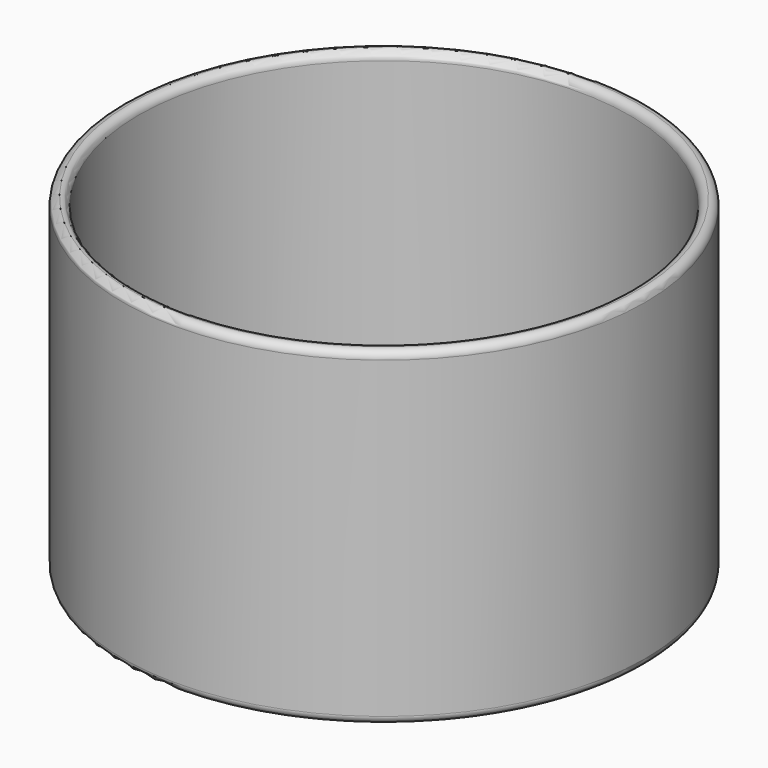
from build123d import *

# Parameters (mm, degrees)
F0_W = 42.2452799976
F0_H = 53.2546564937
F2_T = -2.54
F3_R = 1.26999
F4_R = 1.27


# Not quite as in the source:
# - a fillet or chamfer is up to 0.001 mm smaller than in the source, because OpenCascade refuses the exact size


with BuildPart() as f1:
    # F0 (on Front) → F1 (revolve)
    with BuildSketch(Plane.XZ):
        with Locations((-21.1226399988, 1.152144745)):
            Rectangle(F0_W, F0_H)
    revolve(axis=Axis((0, 0, 1.152144745), (0, 0, 1)))

    # F2
    f2_openings = [f1.faces().sort_by_distance(p)[0] for p in [
        (0, 0, 27.779473),
    ]]
    offset(amount=F2_T, openings=f2_openings)

    # F3 (radius 1.27 in the source; OpenCascade refuses exactly that, so slightly less here)
    f3_edges = [f1.edges().sort_by_distance(p)[0] for p in [
        (39.70528, 0, 27.779473),
        (42.24528, 0, 27.779473),
    ]]
    fillet(f3_edges, radius=F3_R)

    # F4
    f4_edges = [f1.edges().sort_by_distance(p)[0] for p in [
        (39.70528, 0, -22.935184),
        (42.24528, 0, -25.475184),
    ]]
    fillet(f4_edges, radius=F4_R)


solid = f1.part
